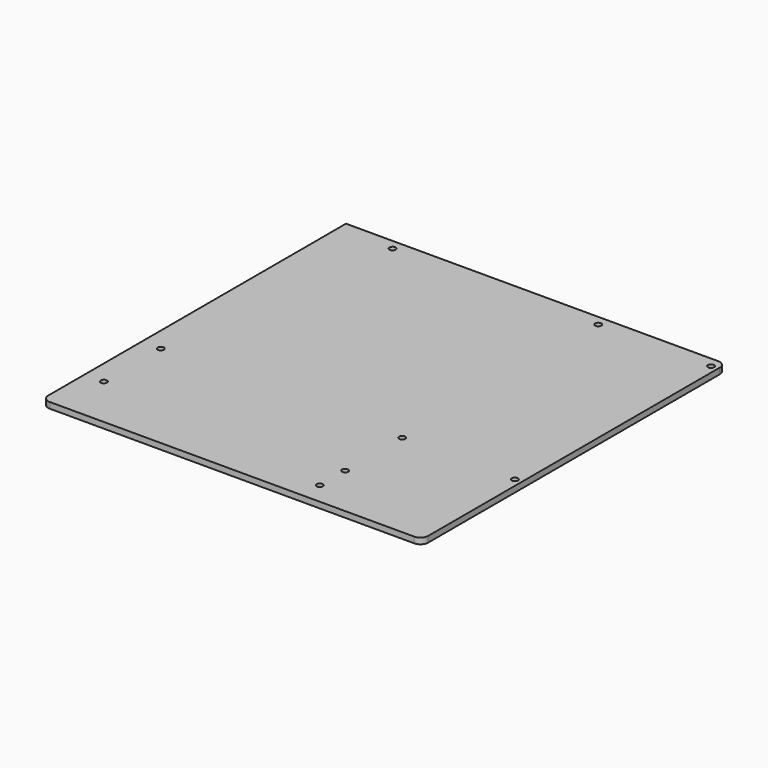
from build123d import *

# Parameters (mm, degrees)
F0_R     = 1.98
F0_W     = 103.5421602428
F0_H     = 6.8848114461
F0_W_2   = 8.5047781467
F0_H_2   = 22.0043957233
F0_W_3   = 28.3794738352
F0_H_3   = 70.3811049461
F0_W_4   = 42.310371995
F0_H_4   = 43.9875721931
F0_W_5   = 6.8728923798
F0_H_5   = 133.4486082196
F0_W_6   = 70.3811049461
F0_H_6   = 22.2639712095
F0_W_7   = 22.4677734077
F0_H_7   = 158.75
F1_DEPTH = 3.81


# Not quite as in the source:
# - a feature of the source that left no trace in its solid (it failed there, or was rolled back) is left out


with BuildPart() as f1:
    # F0 (on Top) → F1 (new body)
    with BuildSketch(Plane.XY):
        with BuildLine():
            ThreePointArc((0, 5), (1.4644660941, 1.4644660941), (5, 0))
            Line((5, 0), (239, 0))
            ThreePointArc((239, 0), (242.5355339059, 1.4644660941), (244, 5))
            Line((244, 5), (244, 239))
            ThreePointArc((244, 239), (242.5355339059, 242.5355339059), (239, 244))
            Line((239, 244), (155.4765701294, 244))
            Line((155.4765701294, 244), (155.4765701294, 221.7360287905))
            Line((155.4765701294, 221.7360287905), (85.0954651833, 221.7360287905))
            Line((85.0954651833, 221.7360287905), (85.0954651833, 244))
            Line((85.0954651833, 244), (22.4677734077, 244))
            Line((22.4677734077, 244), (22.4677734077, 85.25))
            Line((22.4677734077, 85.25), (0, 85.25))
            Line((0, 85.25), (0, 5))
        make_face()
        with Locations((12.27, 34.29)):
            Circle(F0_R, mode=Mode.SUBTRACT)
        with Locations((94.4036040455, 18.8242988661)):
            Rectangle(F0_W, F0_H, mode=Mode.SUBTRACT)
        with Locations((12.27, 80.01)):
            Circle(F0_R, mode=Mode.SUBTRACT)
        with Locations((167.21, 13.97)):
            Circle(F0_R, mode=Mode.SUBTRACT)
        with Locations((167.21, 34.29)):
            Circle(F0_R, mode=Mode.SUBTRACT)
        with Locations((152.7901440859, 81.0341909528)):
            Rectangle(F0_W_2, F0_H_2, mode=Mode.SUBTRACT)
        with Locations((167.21, 80.01)):
            Circle(F0_R, mode=Mode.SUBTRACT)
        with Locations((239.6, 80.01)):
            Circle(F0_R, mode=Mode.SUBTRACT)
        with Locations((56.3754346222, 171.5611219406)):
            Rectangle(F0_W_3, F0_H_3, mode=Mode.SUBTRACT)
        with Locations((35.13, 237.49)):
            Circle(F0_R, mode=Mode.SUBTRACT)
        with Locations((123.8708272576, 159.014120698)):
            Rectangle(F0_W_4, F0_H_4, mode=Mode.SUBTRACT)
        with Locations((180.2064478397, 157.2181545198)):
            Rectangle(F0_W_5, F0_H_5, mode=Mode.SUBTRACT)
        with Locations((189.3064478397, 157.2181545198)):
            Rectangle(F0_W_5, F0_H_5, mode=Mode.SUBTRACT)
        with Locations((198.4064478397, 157.2181545198)):
            Rectangle(F0_W_5, F0_H_5, mode=Mode.SUBTRACT)
        with Locations((207.5064478397, 157.2181545198)):
            Rectangle(F0_W_5, F0_H_5, mode=Mode.SUBTRACT)
        with Locations((167.21, 237.49)):
            Circle(F0_R, mode=Mode.SUBTRACT)
        with Locations((239.6, 237.49)):
            Circle(F0_R, mode=Mode.SUBTRACT)
        with Locations((94.4036040455, 18.8242988661)):
            Rectangle(F0_W, F0_H)
        with Locations((152.7901440859, 81.0341909528)):
            Rectangle(F0_W_2, F0_H_2)
        with Locations((180.2064478397, 157.2181545198)):
            Rectangle(F0_W_5, F0_H_5)
        with Locations((189.3064478397, 157.2181545198)):
            Rectangle(F0_W_5, F0_H_5)
        with Locations((198.4064478397, 157.2181545198)):
            Rectangle(F0_W_5, F0_H_5)
        with Locations((207.5064478397, 157.2181545198)):
            Rectangle(F0_W_5, F0_H_5)
        with Locations((123.8708272576, 159.014120698)):
            Rectangle(F0_W_4, F0_H_4)
        with Locations((56.3754346222, 171.5611219406)):
            Rectangle(F0_W_3, F0_H_3)
        with Locations((120.2860176563, 232.8680143952)):
            Rectangle(F0_W_6, F0_H_6)
        with Locations((11.2338867038, 164.625)):
            Rectangle(F0_W_7, F0_H_7)
    extrude(amount=F1_DEPTH)


solid = f1.part
